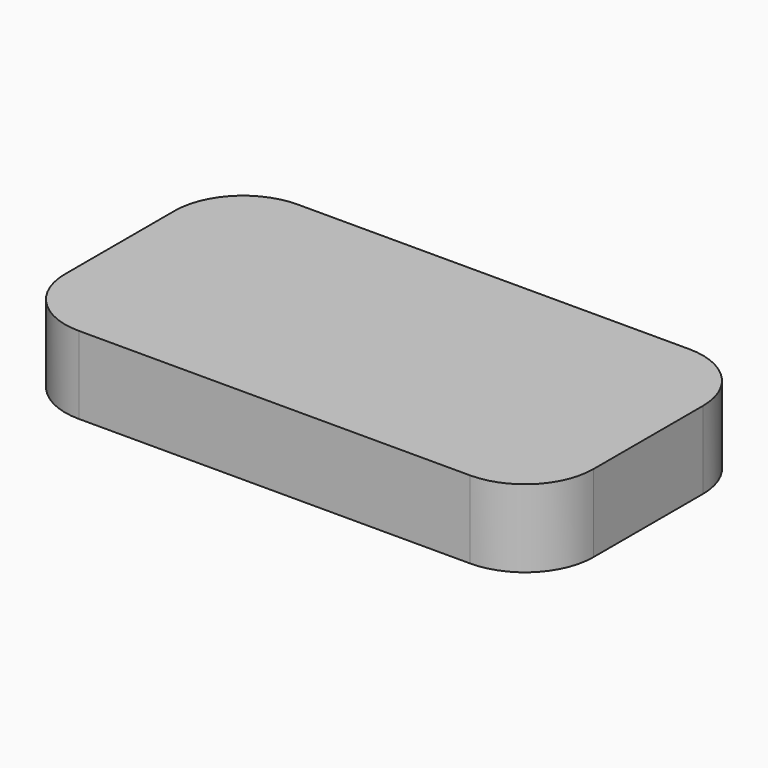
from build123d import *

# Parameters (mm, degrees)
F0_R     = 1.9
F1_DEPTH = 1.7
F2_R     = 1.9
F3_DEPTH = 0.8


# Not quite as in the source:
# - a feature names something its author has since deleted; it is built from what else it names


with BuildPart() as f1:
    # F0 (on Top) → F1 (new body)
    with BuildSketch(Plane.XY):
        with BuildLine():
            Line((-0.3902956496, 3), (-4.2902956496, 3))
            ThreePointArc((-4.2902956496, 3), (-5.3509558214, 2.5606601718), (-5.7902956496, 1.5))
            Line((-5.7902956496, 1.5), (-5.7902956496, -1.5))
            ThreePointArc((-5.7902956496, -1.5), (-5.3509558214, -2.5606601718), (-4.2902956496, -3))
            Line((-4.2902956496, -3), (-0.3902956496, -3))
            Line((-0.3902956496, -3), (0.3902956496, -3))
            Line((0.3902956496, -3), (4.2902956496, -3))
            ThreePointArc((4.2902956496, -3), (5.3509558214, -2.5606601718), (5.7902956496, -1.5))
            Line((5.7902956496, -1.5), (5.7902956496, 1.5))
            ThreePointArc((5.7902956496, 1.5), (5.3509558214, 2.5606601718), (4.2902956496, 3))
            Line((4.2902956496, 3), (0.3902956496, 3))
            Line((0.3902956496, 3), (-0.3902956496, 3))
        make_face()
        with Locations((-2.7, 0)):
            Circle(F0_R, mode=Mode.SUBTRACT)
        with Locations((2.7, 0)):
            Circle(F0_R, mode=Mode.SUBTRACT)
    extrude(amount=F1_DEPTH)

    # F2 (on face) → F3 (join)
    with BuildSketch(Plane.XY.offset(1.7)):
        with BuildLine():
            ThreePointArc((-5.7902956496, -1.5), (-5.3509558214, -2.5606601718), (-4.2902956496, -3))
            Line((-4.2902956496, -3), (4.2902956496, -3))
            ThreePointArc((4.2902956496, -3), (5.3509558214, -2.5606601718), (5.7902956496, -1.5))
            Line((5.7902956496, -1.5), (5.7902956496, 1.5))
            ThreePointArc((5.7902956496, 1.5), (5.3509558214, 2.5606601718), (4.2902956496, 3))
            Line((4.2902956496, 3), (-4.2902956496, 3))
            ThreePointArc((-4.2902956496, 3), (-5.3509558214, 2.5606601718), (-5.7902956496, 1.5))
            Line((-5.7902956496, 1.5), (-5.7902956496, -1.5))
        make_face()
        with Locations((-2.7, 0)):
            Circle(F2_R, mode=Mode.SUBTRACT)
        with Locations((2.7, 0)):
            Circle(F2_R, mode=Mode.SUBTRACT)
        with Locations((-2.7, 0)):
            Circle(F2_R)
        with Locations((2.7, 0)):
            Circle(F2_R)
    extrude(amount=-F3_DEPTH)


solid = f1.part
